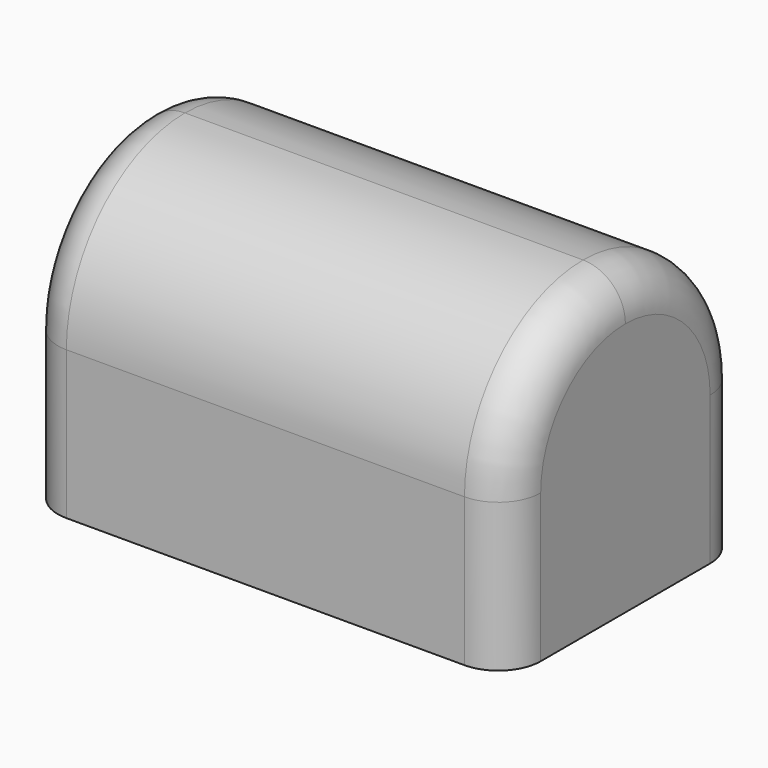
from build123d import *

# Parameters (mm, degrees)
F0_W     = 57
F0_H     = 35
F1_DEPTH = 35
F2_R     = 17.49999
F3_R     = 5


# Not quite as in the source:
# - a fillet or chamfer is up to 0.001 mm smaller than in the source, because OpenCascade refuses the exact size


with BuildPart() as f1:
    # F0 (on Top) → F1 (new body)
    with BuildSketch(Plane.XY):
        Rectangle(F0_W, F0_H)
    extrude(amount=F1_DEPTH)

    # F2 (radius 17.5 in the source; OpenCascade refuses exactly that, so slightly less here)
    f2_edges = [f1.edges().sort_by_distance(p)[0] for p in [
        (0, -17.5, 35),
        (0, 17.5, 35),
    ]]
    fillet(f2_edges, radius=F2_R)

    # F3
    f3_edges = [f1.edges().sort_by_distance(p)[0] for p in [
        (28.5, 17.5, 8.750005),
        (28.5, 12.374372, 29.874372),
        (28.5, -17.5, 8.750005),
        (-28.5, 12.374372, 29.874372),
        (-28.5, -17.5, 8.750005),
        (-28.5, 17.5, 8.750005),
    ]]
    fillet(f3_edges, radius=F3_R)


solid = f1.part
